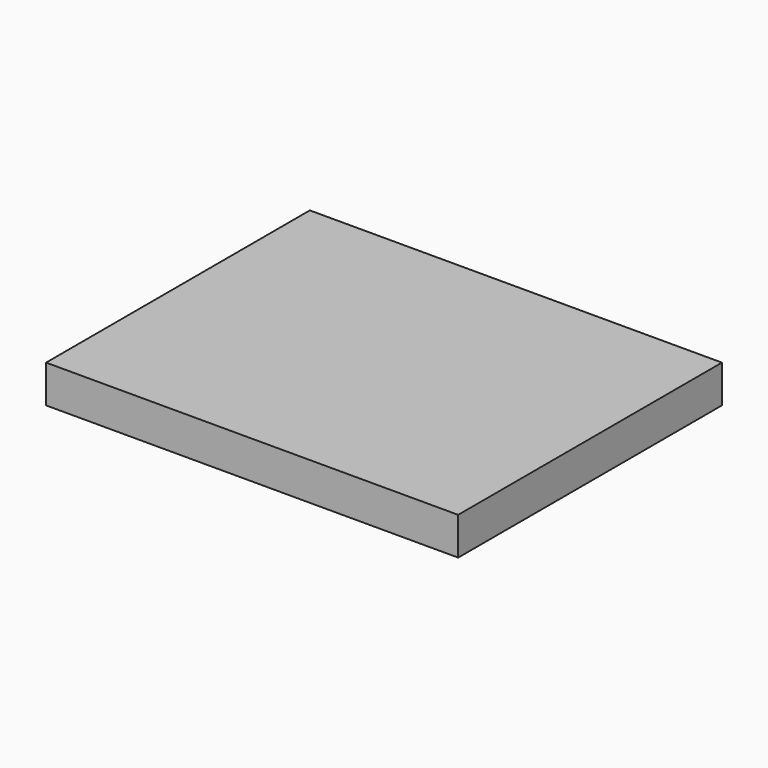
from build123d import *

# Parameters (mm, degrees)
F1_W     = 444.5
F1_H     = 355.6
F2_DEPTH = 40.64


# Not quite as in the source:
# - a variable given as a bare number and used for a length is read in inches; the dataset says mm whatever the document's units were


with BuildPart() as f2:
    # F1 (on Top) → F2 (new body)
    with BuildSketch(Plane.XY):
        Rectangle(F1_W, F1_H)
    extrude(amount=F2_DEPTH)


solid = f2.part
